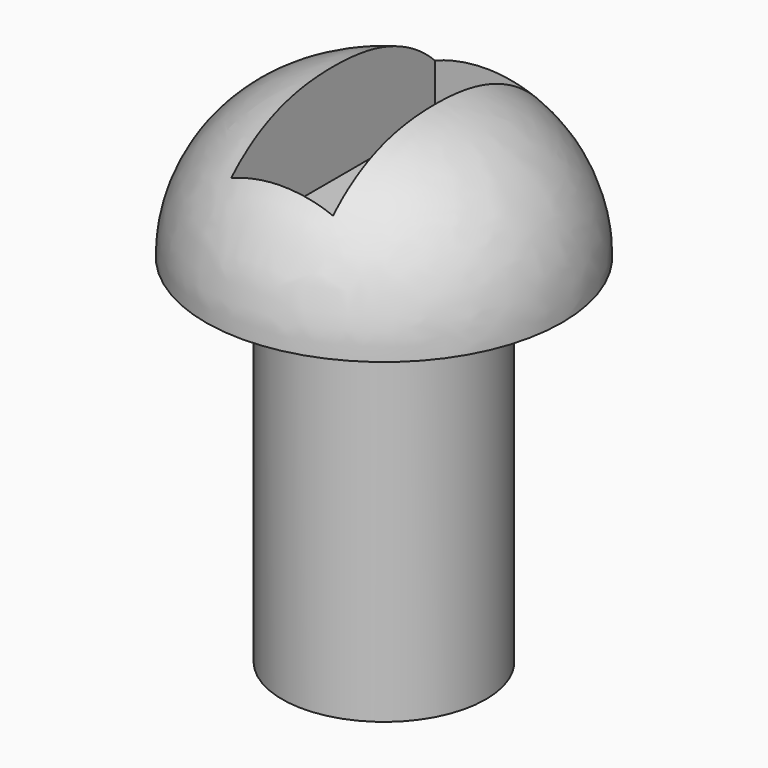
from build123d import *

# Parameters (mm, degrees)
F0_R     = 2.54
F1_DEPTH = 8.89
F2_R     = 4.445
F3_DEPTH = 3.81
F4_W     = 2.54
F4_H     = 6.35
F5_DEPTH = 2.54


# Not quite as in the source:
# - a fillet or chamfer that OpenCascade refuses, or shapes differently, is made with other operations: its cross-section is extruded or revolved along the edge and cut away or added


with BuildPart() as f1:
    # F0 (on Top) → F1 (new body)
    with BuildSketch(Plane.XY):
        Circle(F0_R)
    extrude(amount=F1_DEPTH)

    # F2 (on face) → F3 (join)
    with BuildSketch(Plane.XY.offset(8.89)):
        Circle(F2_R)
    extrude(amount=F3_DEPTH)

    # F4 (on face) → F5 (cut)
    with BuildSketch(Plane.XY.offset(12.7)):
        Rectangle(F4_W, F4_H)
    extrude(amount=-F5_DEPTH, mode=Mode.SUBTRACT)

    # F6: fillet of radius 3.81 on 1 edges, made by hand

    # F6_s1 → F6_t2 (revolve, cut)
    with BuildSketch(Plane.XZ):
        with BuildLine():
            ThreePointArc((4.445, 8.89), (3.3290768363, 11.5840768363), (0.635, 12.7))
            Line((0.635, 12.7), (4.445, 12.7))
            Line((4.445, 12.7), (4.445, 8.89))
        make_face()
    revolve(axis=Axis((0, 0, 12.7), (0, 0, 1)), mode=Mode.SUBTRACT)


solid = f1.part
